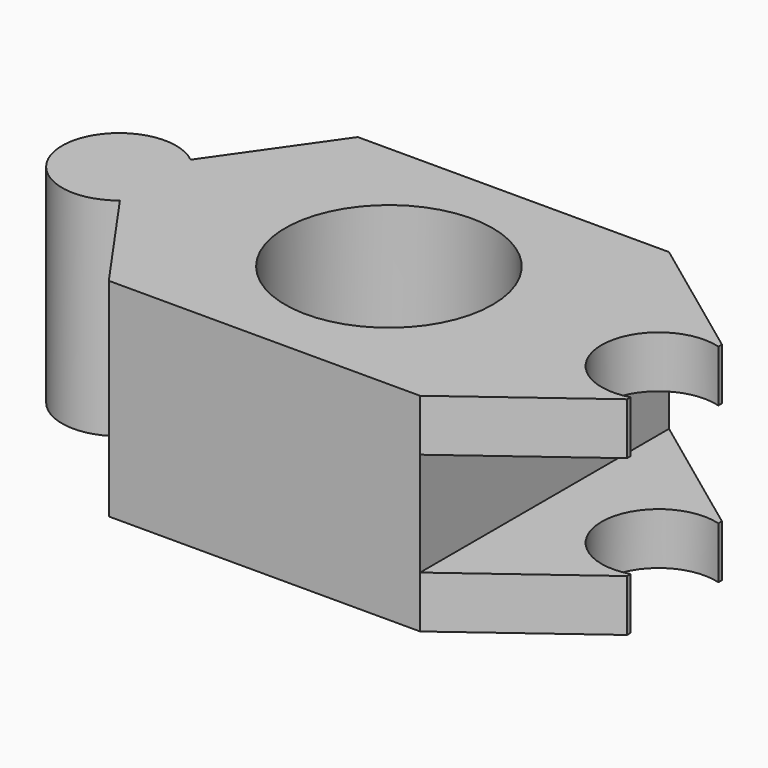
from build123d import *

# Parameters (mm, degrees)
F0_W     = 15
F0_H     = 15
F0_R     = 5
F1_DEPTH = 5
F3_DEPTH = 5
F5_DEPTH = 5
F7_DEPTH = 2.5


with BuildPart() as f1:
    # F0 (on Top) → F1 (new body, symmetric)
    with BuildSketch(Plane.XY):
        Rectangle(F0_W, F0_H)
        Circle(F0_R, mode=Mode.SUBTRACT)
    extrude(amount=F1_DEPTH, both=True)

    # F2 (on Top) → F3 (join, symmetric)
    with BuildSketch(Plane.XY):
        with BuildLine():
            Line((13.7621368783, 2.8581836929), (7.5, 7.5))
            Line((7.5, 7.5), (7.5, -7.5))
            Line((7.5, -7.5), (13.7621368783, -2.8581836929))
            Line((13.7621368783, -2.8581836929), (13.7621368783, -2.6422807153))
            ThreePointArc((13.7621368783, -2.6422807153), (10.25, 0), (13.7621368783, 2.6422807153))
            Line((13.7621368783, 2.6422807153), (13.7621368783, 2.8581836929))
        make_face()
    extrude(amount=F3_DEPTH, both=True)

    # F4 (on Top) → F5 (join, symmetric)
    with BuildSketch(Plane.XY):
        with BuildLine():
            Line((-7.5, 7.5), (-11.2602819583, 2.1297608165))
            ThreePointArc((-11.2602819583, 2.1297608165), (-15.75, 0), (-11.2602819583, -2.1297608165))
            Line((-11.2602819583, -2.1297608165), (-7.5, -7.5))
            Line((-7.5, -7.5), (-7.5, 7.5))
        make_face()
    extrude(amount=F5_DEPTH, both=True)

    # F6 (on Top) → F7 (cut, symmetric)
    with BuildSketch(Plane.XY):
        with BuildLine():
            Line((-7.5, -2.1297608165), (-7.5, 2.1297608165))
            Line((-7.5, 2.1297608165), (-7.5, 7.5))
            Line((-7.5, 7.5), (-11.2602819583, 7.5))
            Line((-11.2602819583, 7.5), (-11.2602819583, 2.1297608165))
            ThreePointArc((-11.2602819583, 2.1297608165), (-10.25, 0), (-11.2602819583, -2.1297608165))
            Line((-11.2602819583, -2.1297608165), (-11.2602819583, -7.5))
            Line((-11.2602819583, -7.5), (-7.5, -7.5))
            Line((-7.5, -7.5), (-7.5, -2.1297608165))
        make_face()
        Polygon((7.5, 7.5), (7.5, 2.8581836929), (7.5, -2.8581836929), (7.5, -7.5), (13.7621368783, -7.5), (13.7621368783, -2.8581836929), (13.7621368783, 2.8581836929), (13.7621368783, 7.5), align=None)
    extrude(amount=F7_DEPTH, both=True, mode=Mode.SUBTRACT)


solid = f1.part
